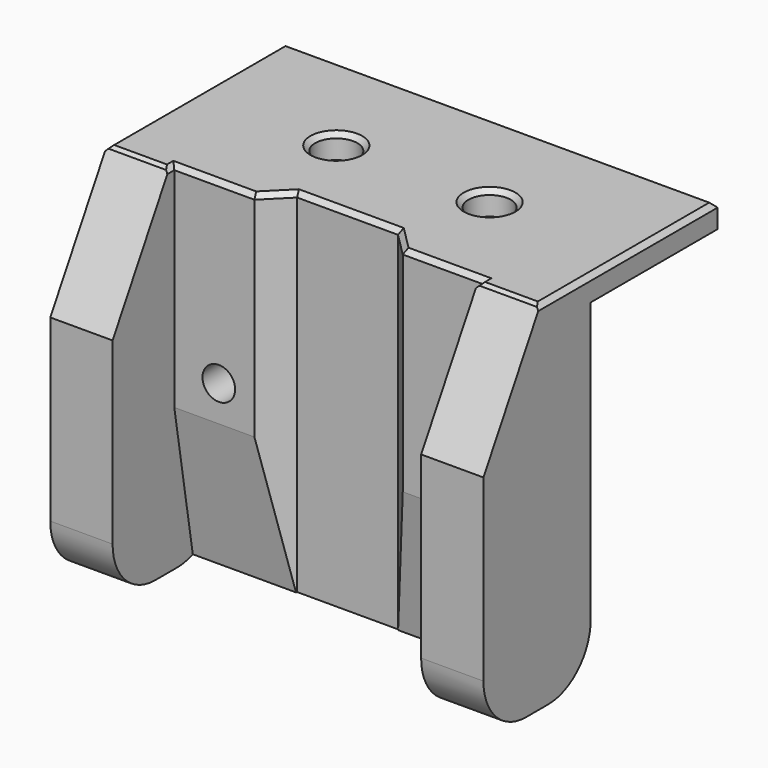
from build123d import *

# Parameters (mm, degrees)
F0_W           = 13.375
F0_H           = 2
F1_DEPTH       = 18.25
F2_R           = 1.7808687455
F2_R_2         = 1.7800904517
F3_DEPTH       = 2
F4_W           = 11.3
F4_H           = 30
F5_DEPTH       = 18.25
F6_W           = 26
F6_H           = 6.5
F7_DEPTH       = 30
F9_DEPTH       = 30
F11_DEPTH      = 13
F11_DEPTH_BACK = 13
F12_R          = 1.375
F13_DEPTH      = 4.8
F14_W          = 5.5
F14_H          = 5.5
F15_DEPTH      = 1.5
F16_T1_DEPTH   = 27.75
F16_T3_DEPTH   = 27.75
F16_T5_DEPTH   = 59
F17_SIZE2      = 10.3923048454
F17_SIZE       = 6
F18_T1_DEPTH   = 20.7323463904
F18_T3_DEPTH   = 6.4746360003
F18_T5_DEPTH   = 38.5573463904
F18_T7_DEPTH   = 1.5286731952
F18_T9_DEPTH   = 7.7786731952
F18_T11_DEPTH  = 6.4746360003
F18_T13_DEPTH  = 7.7786731952
F18_T18_DEPTH  = 4.8857735151
F18_T23_DEPTH  = 10.5573463904
F18_T29_DEPTH  = 4.8857735151
F18_T39_DEPTH  = 2.5573463904
F18_T43_DEPTH  = 8.8073463904
F18_T50_DEPTH  = 4.8857735151
F18_T54_DEPTH  = 10.5573463904
F18_T61_DEPTH  = 2.5573463904
F18_T65_DEPTH  = 8.8073463904
F18_T72_DEPTH  = 10.5573463904
F18_T76_DEPTH  = 4.8857735151


# Not quite as in the source:
# - a fillet or chamfer that OpenCascade refuses, or shapes differently, is made with other operations: its cross-section is extruded or revolved along the edge and cut away or added


with BuildPart() as f1:
    # F0 (on Right) → F1 (new body, symmetric)
    with BuildSketch(Plane.YZ):
        with Locations((6.6875, 1)):
            Rectangle(F0_W, F0_H)
    extrude(amount=F1_DEPTH, both=True)

    # F2 (on face) → F3 (cut, through all)
    with BuildSketch(Plane.XY.offset(2)):
        with Locations((6.5276143141, 4)):
            Circle(F2_R)
        with Locations((-6.3883271068, 4)):
            Circle(F2_R_2)
    extrude(amount=-F3_DEPTH, mode=Mode.SUBTRACT)

    # F4 (on Right) → F5 (join, symmetric)
    with BuildSketch(Plane.YZ):
        with Locations((-5.65, -13)):
            Rectangle(F4_W, F4_H)
    extrude(amount=F5_DEPTH, both=True)

    # F6 (on face) → F7 (cut, through all)
    with BuildSketch(Plane(origin=(0, 0, -28), x_dir=(1, 0, 0), z_dir=(0, 0, -1))):
        with Locations((0, 8.05)):
            Rectangle(F6_W, F6_H)
    extrude(amount=-F7_DEPTH, mode=Mode.SUBTRACT)

    # F8 (on face) → F9 (cut, through all)
    with BuildSketch(Plane(origin=(0, 0, -28), x_dir=(1, 0, 0), z_dir=(0, 0, -1))):
        Polygon((6.25, 4.8), (-6.25, 4.8), (-4.25, 2.8), (4.25, 2.8), align=None)
    extrude(amount=-F9_DEPTH, mode=Mode.SUBTRACT)

    # F10 (on Right) → F11 (cut, two sides)
    with BuildSketch(Plane.YZ) as f11_sk:
        Polygon((-4.8, -28), (-2.8, -28), (-4.8, -16), align=None)
    extrude(amount=F11_DEPTH, mode=Mode.SUBTRACT)
    extrude(f11_sk.sketch, amount=-F11_DEPTH_BACK, mode=Mode.SUBTRACT)

    # F12 (on face) → F13 (cut, through all)
    with BuildSketch(Plane.XZ.offset(4.8)):
        with Locations((-9.25, -13)):
            Circle(F12_R)
        with Locations((9.25, -13)):
            Circle(F12_R)
    extrude(amount=-F13_DEPTH, mode=Mode.SUBTRACT)

    # F14 (on face) → F15 (cut)
    with BuildSketch(Plane(origin=(0, 0, 0), x_dir=(-1, 0, 0), z_dir=(0, 1, 0))):
        with Locations((-9.25, -13)):
            Rectangle(F14_W, F14_H)
        with Locations((9.25, -13)):
            Rectangle(F14_W, F14_H)
    extrude(amount=-F15_DEPTH, mode=Mode.SUBTRACT)

    # F16: fillet of radius 4.5 on 3 edges, made by hand

    # F16_s2 → F16_t1 (cut)
    with BuildSketch(Plane.YZ.offset(-29.5)):
        with BuildLine():
            ThreePointArc((-11.3, -23.5), (-9.9819805153, -26.6819805153), (-6.8, -28))
            Line((-6.8, -28), (-11.3, -28))
            Line((-11.3, -28), (-11.3, -23.5))
        make_face()
    extrude(amount=F16_T1_DEPTH, mode=Mode.SUBTRACT)

    # F16_s4 → F16_t3 (cut)
    with BuildSketch(Plane.YZ.offset(1.75)):
        with BuildLine():
            ThreePointArc((-6.8, -28), (-9.9819805153, -26.6819805153), (-11.3, -23.5))
            Line((-11.3, -23.5), (-11.3, -28))
            Line((-11.3, -28), (-6.8, -28))
        make_face()
    extrude(amount=F16_T3_DEPTH, mode=Mode.SUBTRACT)

    # F16_s6 → F16_t5 (cut)
    with BuildSketch(Plane.YZ.offset(-29.5)):
        with BuildLine():
            ThreePointArc((-4.5, -28), (-1.3180194847, -26.6819805153), (0, -23.5))
            Line((0, -23.5), (0, -28))
            Line((0, -28), (-4.5, -28))
        make_face()
    extrude(amount=F16_T5_DEPTH, mode=Mode.SUBTRACT)

    # F17
    f17_edges = [f1.edges().sort_by_distance(p)[0] for p in [
        (-15.625, -11.3, 2),
        (15.625, -11.3, 2),
    ]]
    f17_side = f1.faces().sort_by_distance((-0.00209, 3.324537, 2))[0]
    chamfer(f17_edges, length=F17_SIZE, length2=F17_SIZE2, reference=f17_side)

    # F18: chamfer of 0.4 on 14 edges, made by hand

    # F18_s2 → F18_t1 (cut)
    with BuildSketch(Plane.XZ.offset(-14.4036731952)):
        Polygon((-18.25, 1.6), (-17.85, 2), (-18.25, 2), align=None)
        Polygon((17.85, 2), (18.25, 1.6), (18.25, 2), align=None)
    extrude(amount=F18_T1_DEPTH, mode=Mode.SUBTRACT)

    # F18_s4 → F18_t3 (cut)
    with BuildSketch(Plane.YZ.offset(-18.8623180002)):
        Polygon((-5.4154700538, 1.8), (-5.0690598923, 2), (-5.3, 2), align=None)
    extrude(amount=F18_T3_DEPTH, mode=Mode.SUBTRACT)

    # F18_s6 → F18_t5 (cut)
    with BuildSketch(Plane.YZ.offset(-19.2786731952)):
        Polygon((12.975, 2), (13.375, 1.6), (13.375, 2), align=None)
    extrude(amount=F18_T5_DEPTH, mode=Mode.SUBTRACT)

    # F18_s8 → F18_t7 (cut)
    with BuildSketch(Plane.XZ.offset(4.8)):
        Polygon((-13.4, 2), (-13, 1.6), (-13, 2), align=None)
        Polygon((13.4, 2), (13, 1.6), (13, 2), align=None)
    extrude(amount=F18_T7_DEPTH, mode=Mode.SUBTRACT)

    # F18_s10 → F18_t9 (cut)
    with BuildSketch(Plane.YZ.offset(-13)):
        Polygon((-4.4, 2), (-4.8, 1.6), (-4.8, 2), align=None)
    extrude(amount=F18_T9_DEPTH, mode=Mode.SUBTRACT)

    # F18_s12 → F18_t11 (cut)
    with BuildSketch(Plane.YZ.offset(12.3876819998)):
        Polygon((-5.0690598923, 2), (-5.4154700538, 1.8), (-5.3, 2), align=None)
    extrude(amount=F18_T11_DEPTH, mode=Mode.SUBTRACT)

    # F18_s14 → F18_t13 (cut)
    with BuildSketch(Plane.YZ.offset(5.2213268048)):
        Polygon((-4.4, 2), (-4.8, 1.6), (-4.8, 2), align=None)
    extrude(amount=F18_T13_DEPTH, mode=Mode.SUBTRACT)


with BuildPart() as f18_tool16:
    # F18_s17 → F18_t18 (new body)
    with BuildSketch(Plane(origin=(-6.2523817919, -6.2523817919, 0), x_dir=(0, 0, 1), z_dir=(0.7071067812, 0.7071067812, 0))):
        Polygon((2, -1.4253048327), (1.6, -1.0253048327), (2, -1.0253048327), align=None)
    extrude(amount=F18_T18_DEPTH)

    split(bisect_by=Plane.XZ.offset(2.8), keep=Keep.TOP)


with BuildPart() as f1_1:
    add(f1.part)

    # F18_t15: cut F18_tool16
    add(f18_tool16.part, mode=Mode.SUBTRACT)


with BuildPart() as f18_tool21:
    # F18_s22 → F18_t23 (new body)
    with BuildSketch(Plane.YZ.offset(-5.2786731952)):
        Polygon((-2.4, 2), (-2.8, 1.6), (-2.8, 2), align=None)
    extrude(amount=F18_T23_DEPTH)

    split(bisect_by=Plane(origin=(-0.725, 0.725, 0), x_dir=(0, 0, 1), z_dir=(0.7071067812, -0.7071067812, 0)), keep=Keep.TOP)

    split(bisect_by=Plane(origin=(0.725, 0.725, 0), x_dir=(0, 0, 1), z_dir=(-0.7071067812, -0.7071067812, 0)), keep=Keep.TOP)


with BuildPart() as f1_2:
    add(f1_1.part)

    # F18_t20: cut F18_tool21
    add(f18_tool21.part, mode=Mode.SUBTRACT)


with BuildPart() as f18_tool27:
    # F18_s28 → F18_t29 (new body)
    with BuildSketch(Plane(origin=(2.7976182081, -2.7976182081, 0), x_dir=(0, 0, 1), z_dir=(0.7071067812, -0.7071067812, 0))):
        Polygon((2, -1.4253048327), (1.6, -1.0253048327), (2, -1.0253048327), align=None)
    extrude(amount=F18_T29_DEPTH)

    split(bisect_by=Plane.XZ.offset(2.8), keep=Keep.TOP)


with BuildPart() as f1_3:
    add(f1_2.part)

    # F18_t26: cut F18_tool27
    add(f18_tool27.part, mode=Mode.SUBTRACT)

    # F18_s31 → F18_t32 (revolve, cut)
    with BuildSketch(Plane.XZ.offset(-4)):
        Polygon((-4.2082366551, 2), (-4.6082366551, 1.6), (-4.6082366551, 2), align=None)
    revolve(axis=Axis((-6.3883271068, 4, 2), (0, 0, 1)), mode=Mode.SUBTRACT)

    # F18_s33 → F18_t34 (revolve, cut)
    with BuildSketch(Plane.XZ.offset(-4)):
        Polygon((8.7084830596, 2), (8.3084830596, 1.6), (8.3084830596, 2), align=None)
    revolve(axis=Axis((6.5276143141, 4, 2), (0, 0, 1)), mode=Mode.SUBTRACT)


with BuildPart() as f18_tool37:
    # F18_s38 → F18_t39 (new body)
    with BuildSketch(Plane.XZ.offset(6.3286731952)):
        Polygon((-13.4, 2), (-13, 1.6), (-13, 2), align=None)
    extrude(amount=-F18_T39_DEPTH)

    split(bisect_by=Plane.XZ.offset(4.8), keep=Keep.BOTTOM)


with BuildPart() as f18_tool41:
    # F18_s42 → F18_t43 (new body)
    with BuildSketch(Plane.YZ.offset(-14.0286731952)):
        Polygon((-4.4, 2), (-4.8, 1.6), (-4.8, 2), align=None)
    extrude(amount=F18_T43_DEPTH)

    split(bisect_by=Plane.YZ.offset(-13), keep=Keep.BOTTOM)


with BuildPart() as f18_tool37_1:
    add(f18_tool37.part)

    # F18_t45: intersect F18_tool41
    add(f18_tool41.part, mode=Mode.INTERSECT)


with BuildPart() as f1_4:
    add(f1_3.part)

    # F18_t35: cut F18_tool37
    add(f18_tool37_1.part, mode=Mode.SUBTRACT)


with BuildPart() as f18_tool48:
    # F18_s49 → F18_t50 (new body)
    with BuildSketch(Plane(origin=(-6.2523817919, -6.2523817919, 0), x_dir=(0, 0, 1), z_dir=(0.7071067812, 0.7071067812, 0))):
        Polygon((2, -1.4253048327), (1.6, -1.0253048327), (2, -1.0253048327), align=None)
    extrude(amount=F18_T50_DEPTH)

    split(bisect_by=Plane.XZ.offset(2.8), keep=Keep.BOTTOM)


with BuildPart() as f18_tool52:
    # F18_s53 → F18_t54 (new body)
    with BuildSketch(Plane.YZ.offset(-5.2786731952)):
        Polygon((-2.4, 2), (-2.8, 1.6), (-2.8, 2), align=None)
    extrude(amount=F18_T54_DEPTH)

    split(bisect_by=Plane(origin=(-0.725, 0.725, 0), x_dir=(0, 0, 1), z_dir=(-0.7071067812, 0.7071067812, 0)), keep=Keep.TOP)


with BuildPart() as f18_tool48_1:
    add(f18_tool48.part)

    # F18_t56: intersect F18_tool52
    add(f18_tool52.part, mode=Mode.INTERSECT)


with BuildPart() as f1_5:
    add(f1_4.part)

    # F18_t46: cut F18_tool48
    add(f18_tool48_1.part, mode=Mode.SUBTRACT)


with BuildPart() as f18_tool59:
    # F18_s60 → F18_t61 (new body)
    with BuildSketch(Plane.XZ.offset(3.7713268048)):
        Polygon((13.4, 2), (13, 1.6), (13, 2), align=None)
    extrude(amount=F18_T61_DEPTH)

    split(bisect_by=Plane.XZ.offset(4.8), keep=Keep.BOTTOM)


with BuildPart() as f18_tool63:
    # F18_s64 → F18_t65 (new body)
    with BuildSketch(Plane.YZ.offset(5.2213268048)):
        Polygon((-4.4, 2), (-4.8, 1.6), (-4.8, 2), align=None)
    extrude(amount=F18_T65_DEPTH)

    split(bisect_by=Plane.YZ.offset(13), keep=Keep.TOP)


with BuildPart() as f18_tool59_1:
    add(f18_tool59.part)

    # F18_t67: intersect F18_tool63
    add(f18_tool63.part, mode=Mode.INTERSECT)


with BuildPart() as f1_6:
    add(f1_5.part)

    # F18_t57: cut F18_tool59
    add(f18_tool59_1.part, mode=Mode.SUBTRACT)


with BuildPart() as f18_tool70:
    # F18_s71 → F18_t72 (new body)
    with BuildSketch(Plane.YZ.offset(-5.2786731952)):
        Polygon((-2.4, 2), (-2.8, 1.6), (-2.8, 2), align=None)
    extrude(amount=F18_T72_DEPTH)

    split(bisect_by=Plane(origin=(0.725, 0.725, 0), x_dir=(0, 0, 1), z_dir=(0.7071067812, 0.7071067812, 0)), keep=Keep.TOP)


with BuildPart() as f18_tool74:
    # F18_s75 → F18_t76 (new body)
    with BuildSketch(Plane(origin=(2.7976182081, -2.7976182081, 0), x_dir=(0, 0, 1), z_dir=(0.7071067812, -0.7071067812, 0))):
        Polygon((2, -1.4253048327), (1.6, -1.0253048327), (2, -1.0253048327), align=None)
    extrude(amount=F18_T76_DEPTH)

    split(bisect_by=Plane.XZ.offset(2.8), keep=Keep.BOTTOM)


with BuildPart() as f18_tool70_1:
    add(f18_tool70.part)

    # F18_t78: intersect F18_tool74
    add(f18_tool74.part, mode=Mode.INTERSECT)


with BuildPart() as f1_7:
    add(f1_6.part)

    # F18_t68: cut F18_tool70
    add(f18_tool70_1.part, mode=Mode.SUBTRACT)


solid = f1_7.part
